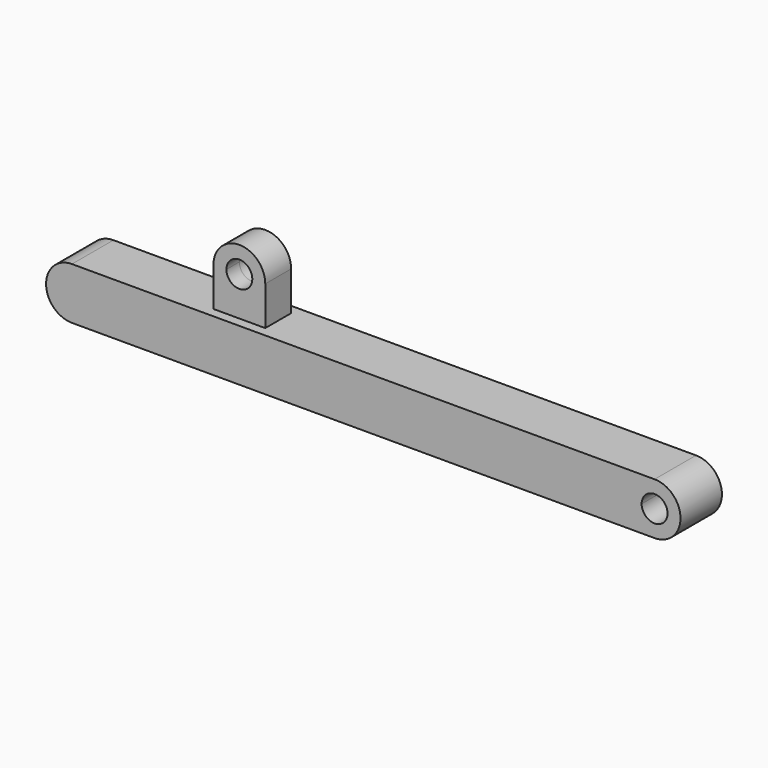
from build123d import *

# Parameters (mm, degrees)
F0_W     = 20
F0_H     = 20
F1_DEPTH = 20
F2_DEPTH = 12.5
F3_D     = 20
F3_DEPTH = 20.001
F4_D     = 20


with BuildPart() as f1:
    # F0 (on Front) → F1 (new body, symmetric)
    with BuildSketch(Plane.XZ):
        with BuildLine():
            ThreePointArc((-115.6540289521, -20), (-101.5118933284, -14.1421356237), (-95.6540289521, 0))
            Line((-95.6540289521, 0), (-115.6540289521, 0))
            Line((-115.6540289521, 0), (-135.6540289521, 0))
            ThreePointArc((-135.6540289521, 0), (-129.7961645759, -14.1421356237), (-115.6540289521, -20))
        make_face()
        with BuildLine():
            Line((-95.6540289521, 20), (-95.6540289521, 0))
            ThreePointArc((-95.6540289521, 0), (-101.5118933284, -14.1421356237), (-115.6540289521, -20))
            Line((-115.6540289521, -20), (211.0609319716, -20))
            ThreePointArc((211.0609319716, -20), (231.0609319716, 0), (211.0609319716, 20))
            Line((211.0609319716, 20), (-95.6540289521, 20))
        make_face()
        with Locations((-105.6540289521, 10)):
            Rectangle(F0_W, F0_H)
        with Locations((-125.6540289521, 10)):
            Rectangle(F0_W, F0_H)
        with BuildLine():
            Line((-238.9390680284, -20), (-115.6540289521, -20))
            ThreePointArc((-115.6540289521, -20), (-129.7961645759, -14.1421356237), (-135.6540289521, 0))
            Line((-135.6540289521, 0), (-135.6540289521, 20))
            Line((-135.6540289521, 20), (-238.9390680284, 20))
            ThreePointArc((-238.9390680284, 20), (-258.9390680284, 0), (-238.9390680284, -20))
        make_face()
    extrude(amount=F1_DEPTH, both=True)

    # F0 (on Front) → F2 (join, symmetric)
    with BuildSketch(Plane.XZ):
        with BuildLine():
            ThreePointArc((-115.6540289521, -20), (-101.5118933284, -14.1421356237), (-95.6540289521, 0))
            Line((-95.6540289521, 0), (-115.6540289521, 0))
            Line((-115.6540289521, 0), (-135.6540289521, 0))
            ThreePointArc((-135.6540289521, 0), (-129.7961645759, -14.1421356237), (-115.6540289521, -20))
        make_face()
        with BuildLine():
            Line((-95.6540289521, 20), (-95.6540289521, 0))
            ThreePointArc((-95.6540289521, 0), (-101.5118933284, -14.1421356237), (-115.6540289521, -20))
            Line((-115.6540289521, -20), (211.0609319716, -20))
            ThreePointArc((211.0609319716, -20), (231.0609319716, 0), (211.0609319716, 20))
            Line((211.0609319716, 20), (-95.6540289521, 20))
        make_face()
        with Locations((-105.6540289521, 10)):
            Rectangle(F0_W, F0_H)
        with Locations((-125.6540289521, 10)):
            Rectangle(F0_W, F0_H)
        with BuildLine():
            Line((-238.9390680284, -20), (-115.6540289521, -20))
            ThreePointArc((-115.6540289521, -20), (-129.7961645759, -14.1421356237), (-135.6540289521, 0))
            Line((-135.6540289521, 0), (-135.6540289521, 20))
            Line((-135.6540289521, 20), (-238.9390680284, 20))
            ThreePointArc((-238.9390680284, 20), (-258.9390680284, 0), (-238.9390680284, -20))
        make_face()
        with BuildLine():
            Line((-115.6540289521, 20), (-95.6540289521, 20))
            Line((-95.6540289521, 20), (-95.6540289521, 50.1140356064))
            ThreePointArc((-95.6540289521, 50.1140356064), (-115.6540289521, 70.1140356064), (-135.6540289521, 50.1140356064))
            Line((-135.6540289521, 50.1140356064), (-135.6540289521, 20))
            Line((-135.6540289521, 20), (-115.6540289521, 20))
        make_face()
    extrude(amount=F2_DEPTH, both=True)

    # F3 (through all, one way)
    with BuildSketch(Plane(origin=(0, 0, 0), x_dir=(1, 0, 0), z_dir=(0, 1, 0))):
        with Locations((211.0609319716, 0), (-115.6540289521, -50.1140356064)):
            Circle(F3_D / 2)
    extrude(amount=-F3_DEPTH, mode=Mode.SUBTRACT)

    # F4 (through all)
    with Locations(Plane.XZ):
        with Locations((-115.6540289521, 50.1140356064), (211.0609319716, 0)):
            Hole(F4_D / 2)


solid = f1.part
